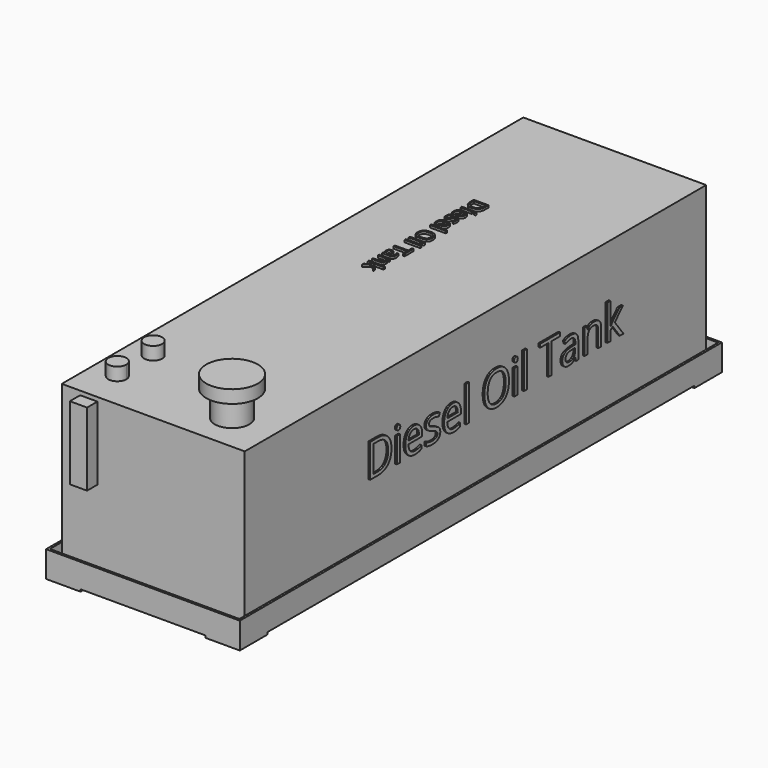
from build123d import *

# Parameters (mm, degrees)
F0_W          = 425
F0_H          = 380
F1_DEPTH      = 1340
F2_W          = 450
F2_H          = 1400
F2_W_2        = 425
F2_H_2        = 1340
F3_DEPTH      = 6
F4_W          = 450
F4_H          = 1400
F4_W_2        = 440
F4_H_2        = 1390
F5_DEPTH      = 50
F6_W          = 40
F6_H          = 170
F7_DEPTH      = 30
F8_R          = 40
F9_DEPTH      = 60
F10_DEPTH     = 30
F8_TEXT_SIZE  = 48.0386487165
F11_DEPTH     = 5
F12_R         = 60
F12_R_2       = 40
F13_DEPTH     = 30
F14_W         = 80
F14_H         = 80
F15_DEPTH     = 5
F16_TEXT_SIZE = 108.520541754
F17_DEPTH     = 4


# Not quite as in the source:
# - Text() gives the source's letters only with a copy of the font that has no kerning and outlines rounded to 1/6400 em; it was checked with that copy


with BuildPart() as f1:
    # F0 (on Front) → F1 (new body)
    with BuildSketch(Plane.XZ):
        with Locations((212.5, 190)):
            Rectangle(F0_W, F0_H)
    extrude(amount=-F1_DEPTH)

    # F2 (on face) → F3 (join)
    with BuildSketch(Plane(origin=(0, 0, 0), x_dir=(1, 0, 0), z_dir=(0, 0, -1))):
        with Locations((212.5, -670)):
            Rectangle(F2_W, F2_H)
        with Locations((212.5, -670)):
            Rectangle(F2_W_2, F2_H_2, mode=Mode.SUBTRACT)
        with Locations((212.5, -670)):
            Rectangle(F2_W_2, F2_H_2)
    extrude(amount=F3_DEPTH)

    # F4 (on face) → F5 (join)
    with BuildSketch(Plane.XY):
        with Locations((212.5, 670)):
            Rectangle(F4_W, F4_H)
        with Locations((212.5, 670)):
            Rectangle(F4_W_2, F4_H_2, mode=Mode.SUBTRACT)
    extrude(amount=F5_DEPTH)

    # F6 (on face) → F7 (join)
    with BuildSketch(Plane.XZ):
        with Locations((62.6989039779, 285.5376815796)):
            Rectangle(F6_W, F6_H)
    extrude(amount=F7_DEPTH)

    # F8 (on face) → F9 (join)
    with BuildSketch(Plane.XY.offset(380)):
        with Locations((325.0986337662, 88.0740657449)):
            Circle(F8_R)
    extrude(amount=F9_DEPTH)

    # F8 (on face) → F10 (join)
    with BuildSketch(Plane.XY.offset(380)):
        with BuildLine():
            ThreePointArc((80.4247952104, 191.0568028688), (44.5755528054, 205.9060452738), (59.4247952104, 170.0568028688))
            ThreePointArc((59.4247952104, 170.0568028688), (74.2740376153, 176.2075604639), (80.4247952104, 191.0568028688))
        make_face()
        with BuildLine():
            ThreePointArc((59.4247952104, 107.9365930557), (44.5755528054, 72.0873506508), (80.4247952104, 86.9365930557))
            ThreePointArc((80.4247952104, 86.9365930557), (74.2740376153, 101.7858354606), (59.4247952104, 107.9365930557))
        make_face()
    extrude(amount=F10_DEPTH)

    # F8 (on face) → F11 (join)
    with BuildSketch(Plane.XY.offset(380)):
        with BuildLine():
            ThreePointArc((59.4247952104, 107.9365930557), (44.5755528054, 72.0873506508), (80.4247952104, 86.9365930557))
            ThreePointArc((80.4247952104, 86.9365930557), (74.2740376153, 101.7858354606), (59.4247952104, 107.9365930557))
        make_face()
        with BuildLine():
            ThreePointArc((80.4247952104, 191.0568028688), (44.5755528054, 205.9060452738), (59.4247952104, 170.0568028688))
            ThreePointArc((59.4247952104, 170.0568028688), (74.2740376153, 176.2075604639), (80.4247952104, 191.0568028688))
        make_face()
        with Locations((325.0986337662, 88.0740657449)):
            Circle(F8_R)
        with Locations(Location((137.7631242778, 1028.4524796512), (0, 0, -89.8216209195))):
            Text('Diesel Oil Tank', F8_TEXT_SIZE, font='Open Sans', text_align=(TextAlign.LEFT, TextAlign.BOTTOM))
    extrude(amount=F11_DEPTH)

    # F12 (on face) → F13 (join)
    with BuildSketch(Plane.XY.offset(440)):
        with Locations((325.0986337662, 88.0740657449)):
            Circle(F12_R)
        with Locations((325.0986337662, 88.0740657449)):
            Circle(F12_R_2, mode=Mode.SUBTRACT)
        with Locations((325.0986337662, 88.0740657449)):
            Circle(F12_R_2)
    extrude(amount=F13_DEPTH)

    # F14 (on face) → F15 (join)
    with BuildSketch(Plane(origin=(0, 0, -6), x_dir=(1, 0, 0), z_dir=(0, 0, -1))):
        with Locations((397.5, -10)):
            Rectangle(F14_W, F14_H)
        with Locations((397.5, -1330)):
            Rectangle(F14_W, F14_H)
        with Locations((27.5, -1330)):
            Rectangle(F14_W, F14_H)
        with Locations((27.5, -10)):
            Rectangle(F14_W, F14_H)
    extrude(amount=F15_DEPTH)

    # F16 (on face) → F17 (join)
    with BuildSketch(Plane.YZ.offset(425)):
        with Locations((348.5294878483, 177.093192935)):
            Text('Diesel Oil Tank', F16_TEXT_SIZE, font='Open Sans', text_align=(TextAlign.LEFT, TextAlign.BOTTOM))
    extrude(amount=F17_DEPTH)


solid = f1.part
